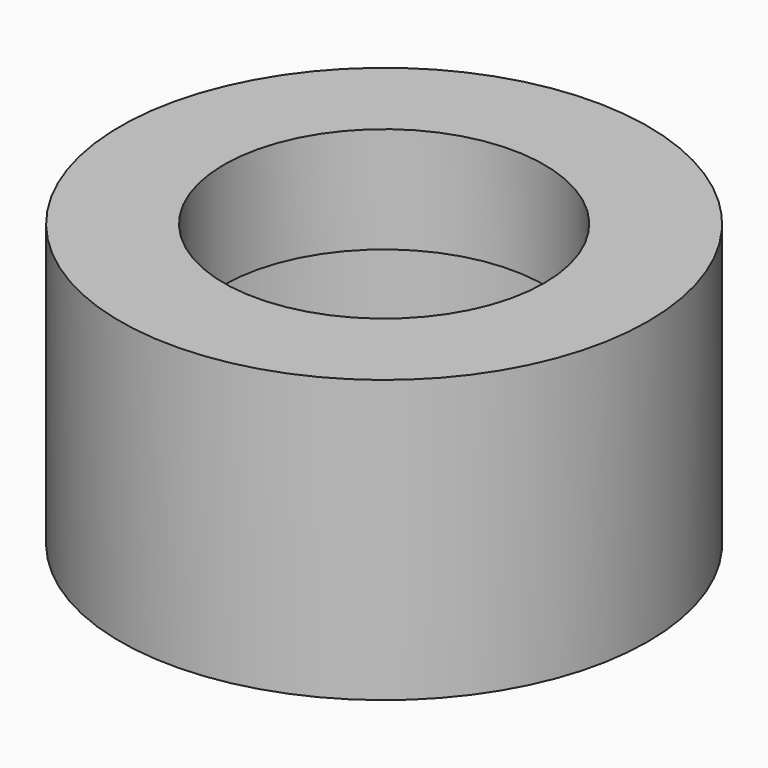
from build123d import *

# Parameters (mm, degrees)
F1_R     = 38.1
F2_DEPTH = 15.2828320861
F3_R     = 23.1262571724
F4_DEPTH = 25.4
F5_R     = 38.1
F5_R_2   = 31.75
F6_DEPTH = 25.4


# Not quite as in the source:
# - a feature names something its author has since deleted; it is built from what else it names


with BuildPart() as f2:
    # F1 (on offset) → F2 (new body)
    with BuildSketch(Plane.XY.offset(-83.2833182067)):
        Circle(F1_R)
    extrude(amount=-F2_DEPTH)

    # F3 (on face) → F4 (cut)
    with BuildSketch(Plane.XY.offset(-83.2833182067)):
        Circle(F3_R)
    extrude(amount=-F4_DEPTH, mode=Mode.SUBTRACT)

    # F5 (on face) → F6 (join)
    with BuildSketch(Plane(origin=(0, 0, -98.5661502928), x_dir=(1, 0, 0), z_dir=(0, 0, -1))):
        Circle(F5_R)
        Circle(F5_R_2, mode=Mode.SUBTRACT)
    extrude(amount=F6_DEPTH)


solid = f2.part
